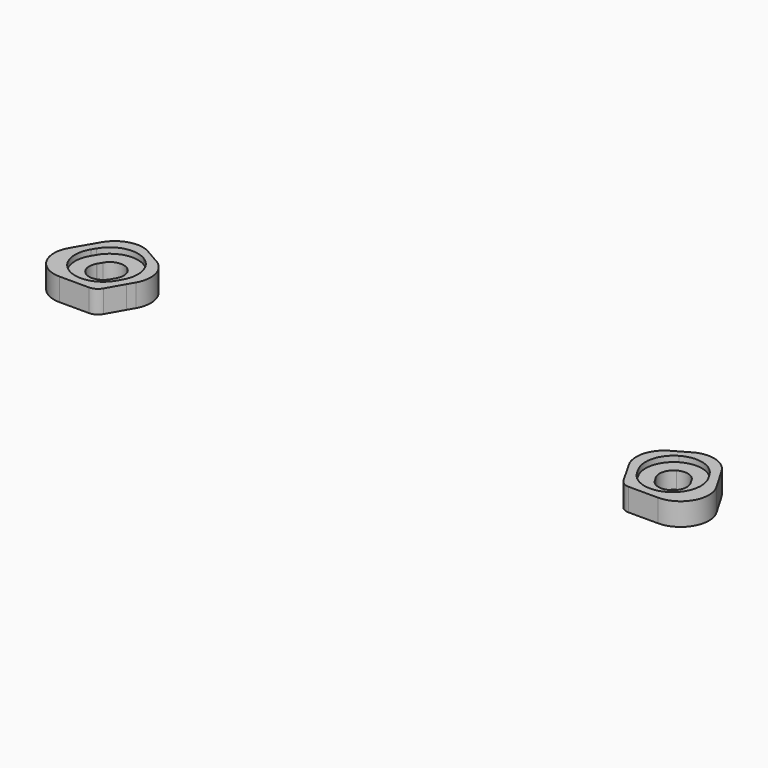
from build123d import *

# Parameters (mm, degrees)
F1_DEPTH = 3
F2_DEPTH = 4


# Not quite as in the source:
# - a feature of the source that left no trace in its solid (it failed there, or was rolled back) is left out


with BuildPart() as f1:
    # F0 (on Top) → F1 (new body)
    with BuildSketch(Plane.XY):
        with BuildLine():
            Line((-45.9526433684, -119.4173828764), (-45.5681720757, -118.7312487792))
            ThreePointArc((-45.5681720757, -118.7312487792), (-45.063382941, -114.9422867004), (-47.382754767, -111.9039384587))
            ThreePointArc((-47.382754767, -111.9039384587), (-51.1733291767, -111.4114028263), (-54.204162304, -113.74058643))
            Line((-54.204162304, -113.74058643), (-54.606684435, -114.4162891074))
            ThreePointArc((-54.606684435, -114.4162891074), (-55.2070897412, -118.268307011), (-52.8591895991, -121.3805238068))
            ThreePointArc((-52.8591895991, -121.3805238068), (-48.9903690941, -121.8608948729), (-45.9526433684, -119.4173828764))
        make_face()
        with BuildLine():
            ThreePointArc((-48.1986328556, -118.3121961967), (-49.7169013888, -119.4679619999), (-51.608311622, -119.2159674351))
            ThreePointArc((-51.608311622, -119.2159674351), (-52.7710236039, -117.703011792), (-52.5277001335, -115.8104665166))
            ThreePointArc((-52.5277001335, -115.8104665166), (-52.5219900166, -115.8005330863), (-52.5162344341, -115.7906259301))
            Line((-52.5162344341, -115.7906259301), (-52.0547569365, -114.9920715737))
            ThreePointArc((-52.0547569365, -114.9920715737), (-50.5360911765, -113.8194261615), (-48.6336124708, -114.0684597488))
            ThreePointArc((-48.6336124708, -114.0684597488), (-47.4679395113, -115.5924838645), (-47.7256896586, -117.4938012538))
            Line((-47.7256896586, -117.4938012538), (-48.1871671562, -118.2923556102))
            ThreePointArc((-48.1871671562, -118.2923556102), (-48.1928772732, -118.3022890405), (-48.1986328556, -118.3121961967))
        make_face(mode=Mode.SUBTRACT)
    extrude(amount=F1_DEPTH)

    # F0 (on Top) → F2 (join)
    with BuildSketch(Plane.XY):
        with BuildLine():
            Line((-44.9889898264, -111.7881834274), (-48.4776615988, -109.7721108748))
            ThreePointArc((-48.4776615988, -109.7721108748), (-52.0379556259, -109.5891437921), (-54.8151657439, -111.8243785613))
            Line((-54.8151657439, -111.8243785613), (-57.2412191282, -115.9784297334))
            ThreePointArc((-57.2412191282, -115.9784297334), (-57.2599668976, -120.989191502), (-52.9236175497, -123.5))
            Line((-52.9236175497, -123.5), (-47.7342220294, -123.5))
            ThreePointArc((-47.7342220294, -123.5), (-46.7306063846, -123.2299582762), (-45.9980088385, -122.4927556374))
            Line((-45.9980088385, -122.4927556374), (-45.9907136957, -122.4799972882))
            Line((-45.9907136957, -122.4799972882), (-44.2837898974, -119.4947877334))
            Line((-44.2837898974, -119.4947877334), (-43.6028383647, -118.3038833569))
            ThreePointArc((-43.6028383647, -118.3038833569), (-43.0528160814, -114.7815764423), (-44.9889898264, -111.7881834274))
        make_face()
        with BuildLine():
            ThreePointArc((-47.382754767, -111.9039384587), (-45.063382941, -114.9422867004), (-45.5681720757, -118.7312487792))
            Line((-45.5681720757, -118.7312487792), (-45.9526433684, -119.4173828764))
            ThreePointArc((-45.9526433684, -119.4173828764), (-48.9903690941, -121.8608948729), (-52.8591895991, -121.3805238068))
            ThreePointArc((-52.8591895991, -121.3805238068), (-55.2070897412, -118.268307011), (-54.606684435, -114.4162891074))
            Line((-54.606684435, -114.4162891074), (-54.204162304, -113.74058643))
            ThreePointArc((-54.204162304, -113.74058643), (-51.1733291767, -111.4114028263), (-47.382754767, -111.9039384587))
        make_face(mode=Mode.SUBTRACT)
    extrude(amount=F2_DEPTH)


with BuildPart() as f1b:
    # F0 (on Top) → F1, piece 2 (new body)
    with BuildSketch(Plane.XY):
        with BuildLine():
            ThreePointArc((47.382754767, -111.9039384587), (45.063382941, -114.9422867004), (45.5681720757, -118.7312487792))
            Line((45.5681720757, -118.7312487792), (45.9526433684, -119.4173828764))
            ThreePointArc((45.9526433684, -119.4173828764), (48.9903690941, -121.8608948729), (52.8591895991, -121.3805238068))
            ThreePointArc((52.8591895991, -121.3805238068), (55.2070897412, -118.268307011), (54.606684435, -114.4162891074))
            Line((54.606684435, -114.4162891074), (54.204162304, -113.74058643))
            ThreePointArc((54.204162304, -113.74058643), (51.1733291767, -111.4114028263), (47.382754767, -111.9039384587))
        make_face()
        with BuildLine():
            ThreePointArc((48.6336124708, -114.0684597488), (50.5360911765, -113.8194261615), (52.0547569365, -114.9920715737))
            Line((52.0547569365, -114.9920715737), (52.5162344341, -115.7906259301))
            Line((52.5162344341, -115.7906259301), (52.5277001335, -115.8104665166))
            ThreePointArc((52.5277001335, -115.8104665166), (52.7710236039, -117.703011792), (51.608311622, -119.2159674351))
            ThreePointArc((51.608311622, -119.2159674351), (49.7169013888, -119.4679619999), (48.1986328556, -118.3121961967))
            ThreePointArc((48.1986328556, -118.3121961967), (48.1928772732, -118.3022890405), (48.1871671562, -118.2923556102))
            Line((48.1871671562, -118.2923556102), (47.7256896586, -117.4938012538))
            ThreePointArc((47.7256896586, -117.4938012538), (47.4679395113, -115.5924838645), (48.6336124708, -114.0684597488))
        make_face(mode=Mode.SUBTRACT)
    extrude(amount=F1_DEPTH)


with BuildPart() as f2:
    # F0 (on Top) → F2, piece 2 (new body)
    with BuildSketch(Plane.XY):
        with BuildLine():
            ThreePointArc((54.8151657439, -111.8243785613), (52.0379556259, -109.5891437921), (48.4776615988, -109.7721108748))
            Line((48.4776615988, -109.7721108748), (44.9889898264, -111.7881834274))
            ThreePointArc((44.9889898264, -111.7881834274), (43.0528160814, -114.7815764423), (43.6028383647, -118.3038833569))
            Line((43.6028383647, -118.3038833569), (44.2837898974, -119.4947877334))
            Line((44.2837898974, -119.4947877334), (45.9907136957, -122.4799972882))
            Line((45.9907136957, -122.4799972882), (45.9980088385, -122.4927556374))
            ThreePointArc((45.9980088385, -122.4927556374), (46.7306063846, -123.2299582762), (47.7342220294, -123.5))
            Line((47.7342220294, -123.5), (52.9236175497, -123.5))
            ThreePointArc((52.9236175497, -123.5), (57.2599668976, -120.989191502), (57.2412191282, -115.9784297334))
            Line((57.2412191282, -115.9784297334), (54.8151657439, -111.8243785613))
        make_face()
        with BuildLine():
            Line((45.9526433684, -119.4173828764), (45.5681720757, -118.7312487792))
            ThreePointArc((45.5681720757, -118.7312487792), (45.063382941, -114.9422867004), (47.382754767, -111.9039384587))
            ThreePointArc((47.382754767, -111.9039384587), (51.1733291767, -111.4114028263), (54.204162304, -113.74058643))
            Line((54.204162304, -113.74058643), (54.606684435, -114.4162891074))
            ThreePointArc((54.606684435, -114.4162891074), (55.2070897412, -118.268307011), (52.8591895991, -121.3805238068))
            ThreePointArc((52.8591895991, -121.3805238068), (48.9903690941, -121.8608948729), (45.9526433684, -119.4173828764))
        make_face(mode=Mode.SUBTRACT)
    extrude(amount=F2_DEPTH)


solid = Compound([f1.part, f1b.part, f2.part])
